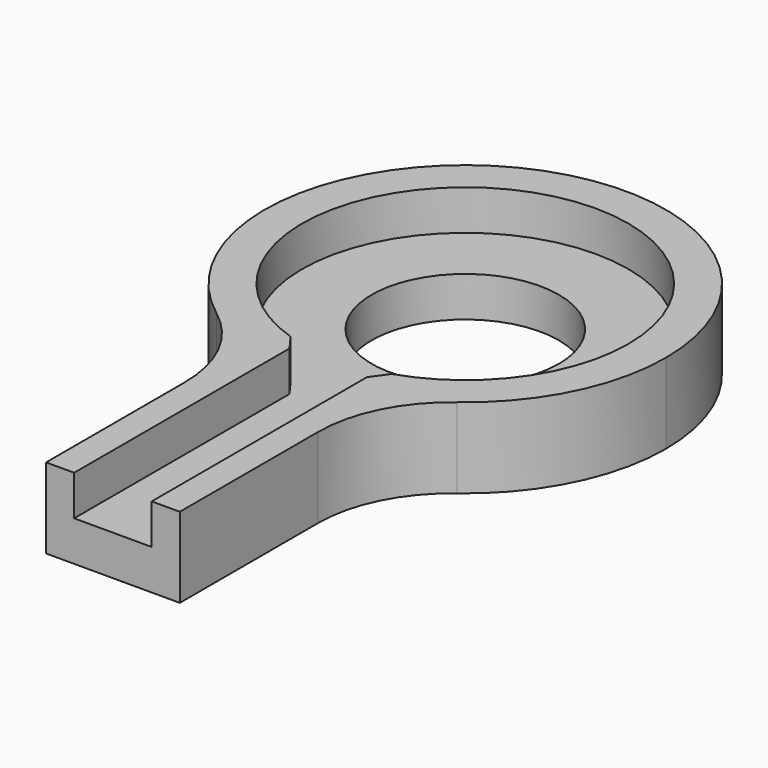
from build123d import *

# Parameters (mm, degrees)
F1_DEPTH    = 3
F3_DEPTH    = 1.5
F4_R        = 3.5
F5_DEPTH    = 1.5
F6_T1_DEPTH = 2.7420993995
F7_R        = 5


# Not quite as in the source:
# - a fillet or chamfer that OpenCascade refuses, or shapes differently, is made with other operations: its cross-section is extruded or revolved along the edge and cut away or added


with BuildPart() as f1:
    # F0 (on Top) → F1 (new body)
    with BuildSketch(Plane.XY):
        with BuildLine():
            ThreePointArc((2.5, -7.0710678119), (6.123724357, -4.3301270189), (7.5, 0))
            ThreePointArc((7.5, 0), (-4.3301270189, 6.123724357), (-2.5, -7.0710678119))
            Line((-2.5, -7.0710678119), (2.5, -7.0710678119))
        make_face()
        with BuildLine():
            Line((2.5, -7.0710678119), (-2.5, -7.0710678119))
            ThreePointArc((-2.5, -7.0710678119), (0, -7.5), (2.5, -7.0710678119))
        make_face()
        with BuildLine():
            ThreePointArc((2.5, -7.0710678119), (0, -7.5), (-2.5, -7.0710678119))
            Line((-2.5, -7.0710678119), (-2.5, -16.4693647414))
            Line((-2.5, -16.4693647414), (2.5, -16.4693647414))
            Line((2.5, -16.4693647414), (2.5, -7.0710678119))
        make_face()
    extrude(amount=F1_DEPTH)

    # F2 (on face) → F3 (cut)
    with BuildSketch(Plane.XY.offset(3)):
        with BuildLine():
            ThreePointArc((1.45, -5.9251582257), (4.79869774, -3.7659660115), (6.1, 0))
            ThreePointArc((6.1, 0), (-3.7659660115, 4.79869774), (-1.45, -5.9251582257))
            Line((-1.45, -5.9251582257), (1.45, -5.9251582257))
        make_face()
        with BuildLine():
            Line((1.45, -5.9251582257), (-1.45, -5.9251582257))
            ThreePointArc((-1.45, -5.9251582257), (0, -6.1), (1.45, -5.9251582257))
        make_face()
        with BuildLine():
            ThreePointArc((1.45, -5.9251582257), (0, -6.1), (-1.45, -5.9251582257))
            Line((-1.45, -5.9251582257), (-1.45, -16.4693647414))
            Line((-1.45, -16.4693647414), (1.45, -16.4693647414))
            Line((1.45, -16.4693647414), (1.45, -5.9251582257))
        make_face()
    extrude(amount=-F3_DEPTH, mode=Mode.SUBTRACT)

    # F4 (on face) → F5 (cut, through all)
    with BuildSketch(Plane.XY.offset(1.5)):
        Circle(F4_R)
    extrude(amount=-F5_DEPTH, mode=Mode.SUBTRACT)

    # F6: chamfer of 0.5 on 2 edges, made by hand

    # F6_s2 → F6_t1 (cut)
    with BuildSketch(Plane.XY.offset(1.5)):
        with BuildLine():
            Line((1.4382509018, -6.4218590468), (1.9014892015, -5.7837185114))
            Line((1.9014892015, -5.7837185114), (1.8983912669, -5.7742104726))
            ThreePointArc((1.8983912669, -5.7742104726), (1.6758695773, -5.854874991), (1.4476229508, -5.9154448516))
            Line((1.4476229508, -5.9154448516), (1.44, -5.9251582257))
            ThreePointArc((1.44, -5.9251582257), (1.44, -6.1735086363), (1.4282509018, -6.4218590468))
            Line((1.4282509018, -6.4218590468), (1.4382509018, -6.4218590468))
        make_face()
        with BuildLine():
            Line((-1.4382509018, -6.4218590468), (-1.9014892015, -5.7837185114))
            Line((-1.9014892015, -5.7837185114), (-1.8983912669, -5.7742104726))
            ThreePointArc((-1.8983912669, -5.7742104726), (-1.6758695773, -5.854874991), (-1.4476229508, -5.9154448516))
            Line((-1.4476229508, -5.9154448516), (-1.44, -5.9251582257))
            ThreePointArc((-1.44, -5.9251582257), (-1.44, -6.1735086363), (-1.4282509018, -6.4218590468))
            Line((-1.4282509018, -6.4218590468), (-1.4382509018, -6.4218590468))
        make_face()
    extrude(amount=F6_T1_DEPTH, mode=Mode.SUBTRACT)

    # F7
    f7_edges = [f1.edges().sort_by_distance(p)[0] for p in [
        (-2.5, -7.071068, 1.5),
        (2.5, -7.071068, 1.5),
    ]]
    fillet(f7_edges, radius=F7_R)


solid = f1.part
